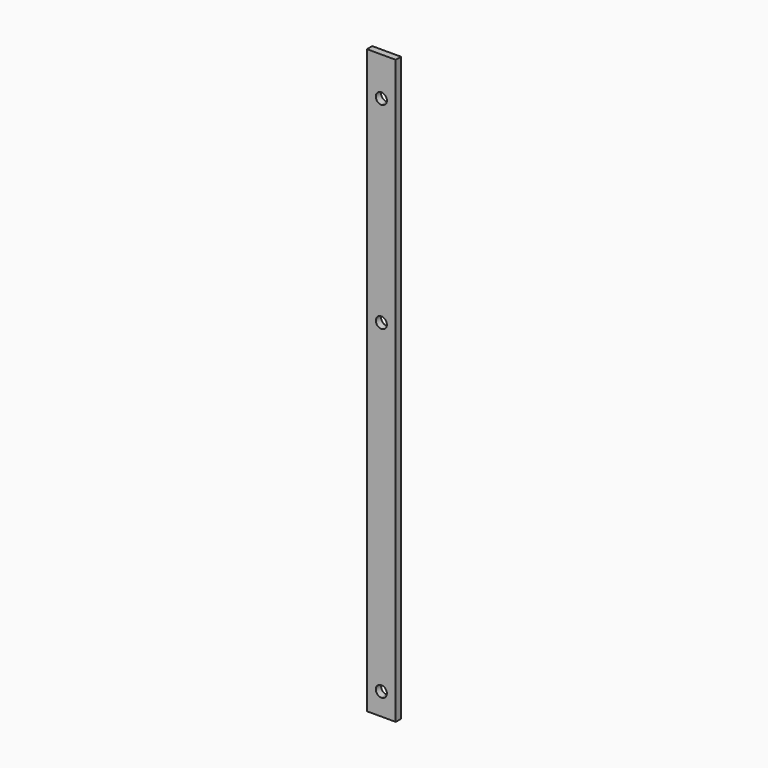
from build123d import *

# Parameters (mm, degrees)
F0_W     = 13
F0_H     = 263
F1_DEPTH = 3
F3_DEPTH = 25


with BuildPart() as f1:
    # F0 (on Front) → F1 (new body)
    with BuildSketch(Plane.XZ):
        Rectangle(F0_W, F0_H)
    extrude(amount=F1_DEPTH)

    # F2 (on face) → F3 (cut)
    with BuildSketch(Plane.XZ.offset(3)):
        with BuildLine():
            ThreePointArc((2.5, 25), (1.767766953, 26.767766953), (0, 27.5))
            ThreePointArc((0, 27.5), (-1.767766953, 23.232233047), (2.5, 25))
        make_face()
        with BuildLine():
            ThreePointArc((2.5, 114), (1.767766953, 115.767766953), (0, 116.5))
            Line((0, 116.5), (0, 114))
            Line((0, 114), (0, 111.5))
            ThreePointArc((0, 111.5), (1.767766953, 112.232233047), (2.5, 114))
        make_face()
        with BuildLine():
            Line((0, 114), (0, 116.5))
            ThreePointArc((0, 116.5), (-2.5, 114), (0, 111.5))
            Line((0, 111.5), (0, 114))
        make_face()
        with BuildLine():
            ThreePointArc((2.5, -121.5), (-1.767766953, -119.732233047), (0, -124))
            ThreePointArc((0, -124), (1.767766953, -123.267766953), (2.5, -121.5))
        make_face()
    extrude(amount=-F3_DEPTH, mode=Mode.SUBTRACT)


solid = f1.part
